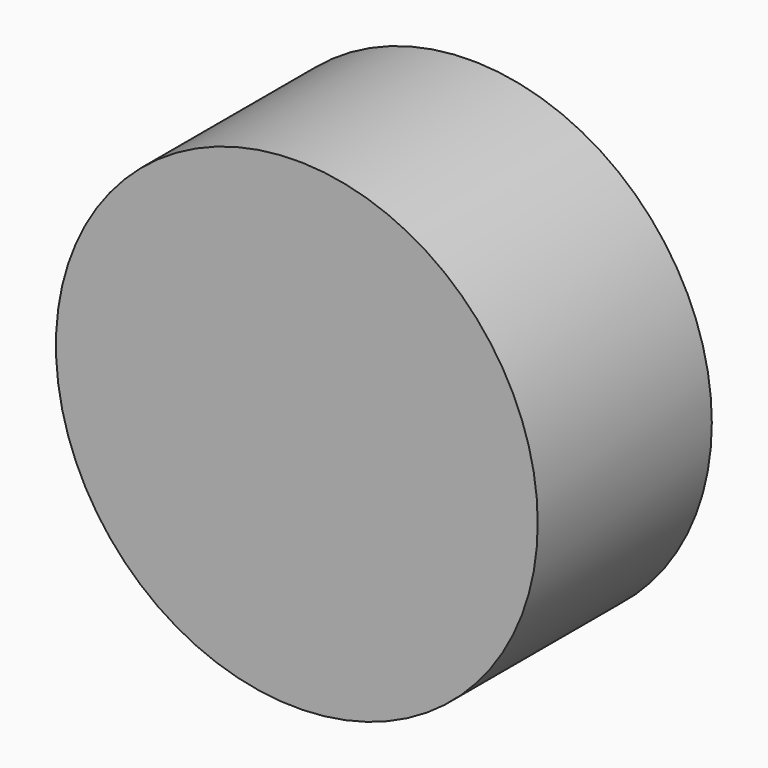
from build123d import *

# Parameters (mm, degrees)
F0_R     = 28.1193476253
F1_DEPTH = 25.4


# Not quite as in the source:
# - the program builds the solid bodies; features that only make, move or delete a surface that nothing else refers to are left out


with BuildPart() as f1:
    # F0 (on Front) → F1 (new body)
    with BuildSketch(Plane.XZ):
        Circle(F0_R)
    extrude(amount=F1_DEPTH)


solid = f1.part
